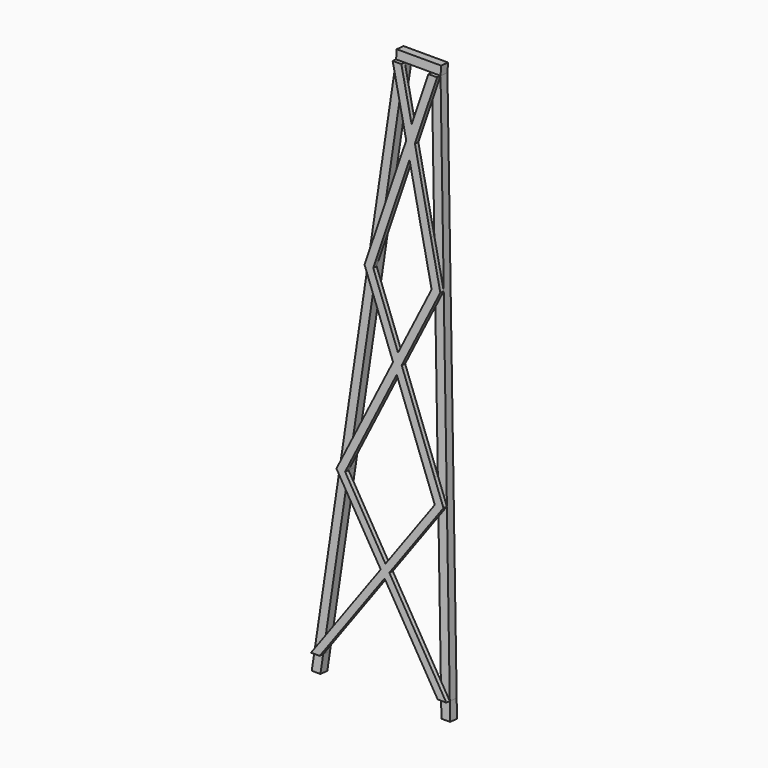
from build123d import *

# Parameters (mm, degrees)
F5_DEPTH = 3.175
F6_DEPTH = 3.175
F7_DEPTH = 1.5875


with BuildPart() as f5:
    # F4 (on line) → F5 (new body)
    with BuildSketch(Plane(origin=(0, -25.2070583861, 2.2053322939), x_dir=(1, 0, 0), z_dir=(0, -0.9961946966, 0.0871557602))):
        Polygon((-8.1596356954, 200.2332657202), (-8.1596356954, 197.0582657202), (-4.9725077112, 197.0582657202), (4.9725077112, 197.0582657202), (8.1596356954, 197.0582657202), (8.1596356954, 200.2332657202), align=None)
    extrude(amount=-F5_DEPTH)


with BuildPart() as f6:
    # F4 (on line) → F6 (new body)
    with BuildSketch(Plane(origin=(0, -25.2070583861, 2.2053322939), x_dir=(1, 0, 0), z_dir=(0, -0.9961946966, 0.0871557602))):
        Polygon((-4.9725077112, 197.0582657202), (-8.1596356954, 197.0582657202), (-5.7162625489, 188.5571090249), align=None)
        Polygon((-5.7162625489, 188.5571090249), (-8.1596356954, 197.0582657202), (-13.9062760659, 131.3738657202), (-9.3244573772, 147.3152534193), align=None)
        Polygon((-9.3244573772, 147.3152534193), (-13.9062760659, 131.3738657202), (-10.7191480817, 131.3738657202), align=None)
        Polygon((-10.7191480817, 131.3738657202), (-13.9062760659, 131.3738657202), (-11.2262337703, 125.5778497774), align=None)
        Polygon((-11.2262337703, 125.5778497774), (-13.9062760659, 131.3738657202), (-19.6529164364, 65.6894657202), (-15.7220336145, 74.1906224154), align=None)
        Polygon((-15.7220336145, 74.1906224154), (-19.6529164364, 65.6894657202), (-16.4657884522, 65.6894657202), align=None)
        Polygon((-16.4657884522, 65.6894657202), (-19.6529164364, 65.6894657202), (-16.8216044507, 61.6224702472), align=None)
        Polygon((-16.8216044507, 61.6224702472), (-19.6529164364, 65.6894657202), (-24.8444469866, 6.35), (-21.1992164113, 11.5861365765), align=None)
        Polygon((-21.1992164113, 11.5861365765), (-24.8444469866, 6.35), (-21.6573190024, 6.35), align=None)
        Polygon((-21.6573190024, 6.35), (-24.8444469866, 6.35), (-25.4, 0), (-22.2370818336, 0), (-22.2128720158, 0), align=None)
    extrude(amount=-F6_DEPTH)


with BuildPart() as f6b:
    # F4 (on line) → F6, piece 2 (new body)
    with BuildSketch(Plane(origin=(0, -25.2070583861, 2.2053322939), x_dir=(1, 0, 0), z_dir=(0, -0.9961946966, 0.0871557602))):
        Polygon((8.1596356954, 197.0582657202), (4.9725077112, 197.0582657202), (5.7162625489, 188.5571090249), align=None)
        Polygon((8.1596356954, 197.0582657202), (5.7162625489, 188.5571090249), (9.3244573772, 147.3152534193), (13.9062760659, 131.3738657202), align=None)
        Polygon((9.3244573772, 147.3152534193), (10.7191480817, 131.3738657202), (13.9062760659, 131.3738657202), align=None)
        Polygon((13.9062760659, 131.3738657202), (10.7191480817, 131.3738657202), (11.2262337703, 125.5778497774), align=None)
        Polygon((19.6529164364, 65.6894657202), (13.9062760659, 131.3738657202), (11.2262337703, 125.5778497774), (15.7220336145, 74.1906224154), align=None)
        Polygon((15.7220336145, 74.1906224154), (16.4657884522, 65.6894657202), (19.6529164364, 65.6894657202), align=None)
        Polygon((19.6529164364, 65.6894657202), (16.4657884522, 65.6894657202), (16.8216044507, 61.6224702472), align=None)
        Polygon((24.8444469866, 6.35), (19.6529164364, 65.6894657202), (16.8216044507, 61.6224702472), (21.1992164113, 11.5861365765), align=None)
        Polygon((21.1992164113, 11.5861365765), (21.6573190024, 6.35), (24.8444469866, 6.35), align=None)
        Polygon((24.8444469866, 6.35), (21.6573190024, 6.35), (22.2128720158, 0), (25.4, 0), align=None)
    extrude(amount=-F6_DEPTH)


with BuildPart() as f7:
    # F4 (on line) → F7 (new body)
    with BuildSketch(Plane(origin=(0, -25.2070583861, 2.2053322939), x_dir=(1, 0, 0), z_dir=(0, -0.9961946966, 0.0871557602))):
        Polygon((-4.9725077112, 197.0582657202), (-8.1596356954, 197.0582657202), (-5.7162625489, 188.5571090249), align=None)
        Polygon((0, 179.7575651368), (-4.9725077112, 197.0582657202), (-5.7162625489, 188.5571090249), (-1.5935639921, 174.213124567), align=None)
        Polygon((5.7162625489, 188.5571090249), (4.9725077112, 197.0582657202), (0, 179.7575651368), (1.5935639921, 174.213124567), align=None)
        Polygon((8.1596356954, 197.0582657202), (4.9725077112, 197.0582657202), (5.7162625489, 188.5571090249), align=None)
        Polygon((1.5935639921, 174.213124567), (0, 179.7575651368), (-1.5935639921, 174.213124567), (0, 168.6686839972), align=None)
        Polygon((-9.3244573772, 147.3152534193), (-10.7191480817, 131.3738657202), (0, 168.6686839972), (-1.5935639921, 174.213124567), align=None)
        Polygon((-9.3244573772, 147.3152534193), (-13.9062760659, 131.3738657202), (-10.7191480817, 131.3738657202), align=None)
        Polygon((1.5935639921, 174.213124567), (0, 168.6686839972), (10.7191480817, 131.3738657202), (9.3244573772, 147.3152534193), align=None)
        Polygon((9.3244573772, 147.3152534193), (10.7191480817, 131.3738657202), (13.9062760659, 131.3738657202), align=None)
        Polygon((10.7191480817, 131.3738657202), (0, 108.1920102412), (1.5935639921, 104.7456757116), (11.2262337703, 125.5778497774), align=None)
        Polygon((13.9062760659, 131.3738657202), (10.7191480817, 131.3738657202), (11.2262337703, 125.5778497774), align=None)
        Polygon((-10.7191480817, 131.3738657202), (-11.2262337703, 125.5778497774), (-1.5935639921, 104.7456757116), (0, 108.1920102412), align=None)
        Polygon((-10.7191480817, 131.3738657202), (-13.9062760659, 131.3738657202), (-11.2262337703, 125.5778497774), align=None)
        Polygon((0, 108.1920102412), (-1.5935639921, 104.7456757116), (0, 101.299341182), (1.5935639921, 104.7456757116), align=None)
        Polygon((-15.7220336145, 74.1906224154), (-16.4657884522, 65.6894657202), (0, 101.299341182), (-1.5935639921, 104.7456757116), align=None)
        Polygon((1.5935639921, 104.7456757116), (0, 101.299341182), (16.4657884522, 65.6894657202), (15.7220336145, 74.1906224154), align=None)
        Polygon((15.7220336145, 74.1906224154), (16.4657884522, 65.6894657202), (19.6529164364, 65.6894657202), align=None)
        Polygon((19.6529164364, 65.6894657202), (16.4657884522, 65.6894657202), (16.8216044507, 61.6224702472), align=None)
        Polygon((16.4657884522, 65.6894657202), (0, 42.0374318105), (1.5935639921, 39.7483808071), (16.8216044507, 61.6224702472), align=None)
        Polygon((-15.7220336145, 74.1906224154), (-19.6529164364, 65.6894657202), (-16.4657884522, 65.6894657202), align=None)
        Polygon((-16.4657884522, 65.6894657202), (-19.6529164364, 65.6894657202), (-16.8216044507, 61.6224702472), align=None)
        Polygon((-16.4657884522, 65.6894657202), (-16.8216044507, 61.6224702472), (-1.5935639921, 39.7483808071), (0, 42.0374318105), align=None)
        Polygon((0, 42.0374318105), (-1.5935639921, 39.7483808071), (0, 37.4593298037), (1.5935639921, 39.7483808071), align=None)
        Polygon((-1.5935639921, 39.7483808071), (-21.1992164113, 11.5861365765), (-21.6573190024, 6.35), (0, 37.4593298037), align=None)
        Polygon((1.5935639921, 39.7483808071), (0, 37.4593298037), (21.6573190024, 6.35), (21.1992164113, 11.5861365765), align=None)
        Polygon((-21.1992164113, 11.5861365765), (-24.8444469866, 6.35), (-21.6573190024, 6.35), align=None)
        Polygon((21.1992164113, 11.5861365765), (21.6573190024, 6.35), (24.8444469866, 6.35), align=None)
    extrude(amount=F7_DEPTH)


solid = Compound([f5.part, f6.part, f6b.part, f7.part])
